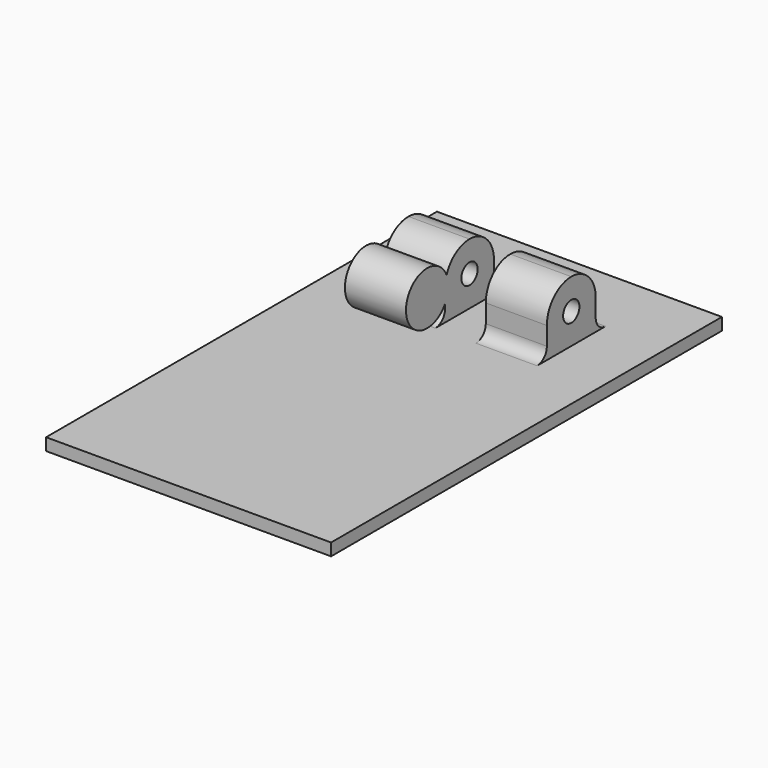
from build123d import *

# Parameters (mm, degrees)
F0_W     = 15
F0_H     = 15
F1_DEPTH = 70
F2_D     = 5
F4_R     = 7.49999
F3_W     = 15
F3_H     = 15
F3_W_2   = 10
F5_DEPTH = 15
F6_R     = 3
F8_DEPTH = 15


# Not quite as in the source:
# - a fillet or chamfer is up to 0.001 mm smaller than in the source, because OpenCascade refuses the exact size


with BuildPart() as f1:
    # F0 (on Right) → F1 (new body)
    with BuildSketch(Plane.YZ):
        with Locations((92.5, 7.5)):
            Rectangle(F0_W, F0_H)
        Polygon((85, 0), (0, 0), (0, -3), (120, -3), (120, 0), (100, 0), align=None)
    extrude(amount=F1_DEPTH)

    # F2 (through all)
    with Locations(Plane(origin=(0, 0, 0), x_dir=(0, 1, 0), z_dir=(-1, 0, 0))):
        with Locations((92.5, -7.5)):
            Hole(F2_D / 2)

    # F4 (radius 7.5 in the source; OpenCascade refuses exactly that, so slightly less here)
    f4_edges = [f1.edges().sort_by_distance(p)[0] for p in [
        (35, 85, 15),
        (35, 100, 15),
    ]]
    fillet(f4_edges, radius=F4_R)

    # F3 (on face) → F5 (cut, through all)
    with BuildSketch(Plane(origin=(0, 100, 0), x_dir=(-1, 0, 0), z_dir=(0, 1, 0))):
        with Locations((-62.5, 7.5)):
            Rectangle(F3_W, F3_H)
        with Locations((-7.5, 7.5)):
            Rectangle(F3_W, F3_H)
        with Locations((-35, 7.5)):
            Rectangle(F3_W_2, F3_H)
    extrude(amount=-F5_DEPTH, mode=Mode.SUBTRACT)

    # F6
    f6_edges = [f1.edges().sort_by_distance(p)[0] for p in [
        (47.5, 85, 0),
        (22.5, 85, 0),
        (22.5, 100, 0),
        (47.5, 100, 0),
    ]]
    fillet(f6_edges, radius=F6_R)

    # F7 (on face) → F8 (join, through all)
    with BuildSketch(Plane.YZ.offset(30)):
        with BuildLine():
            ThreePointArc((85, 7.50001), (85.1162856981, 8.815593818), (85.461536824, 10.0903819596))
            ThreePointArc((85.461536824, 10.0903819596), (73.0188041666, 7.994065349), (85, 4.0358983849))
            Line((85, 4.0358983849), (85, 7.50001))
        make_face()
        with BuildLine():
            ThreePointArc((85, 4.0358983849), (85.7449979984, 5.6972243623), (86, 7.5))
            ThreePointArc((86, 7.5), (85.8639606125, 8.8228776671), (85.461536824, 10.0903819596))
            ThreePointArc((85.461536824, 10.0903819596), (85.1162856981, 8.815593818), (85, 7.50001))
            Line((85, 7.50001), (85, 4.0358983849))
        make_face()
    extrude(amount=-F8_DEPTH)


solid = f1.part
